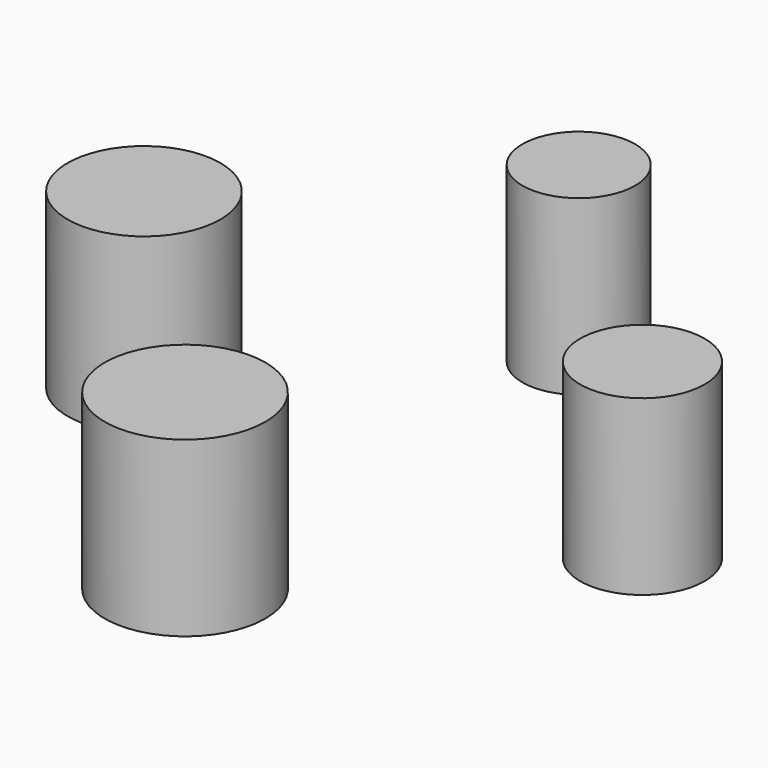
from build123d import *

# Parameters (mm, degrees)
F2_R     = 9.1214460024
F3_DEPTH = 25.4
F4_R     = 11.2110594619
F5_DEPTH = 25.4
F6_R     = 11.7851409997
F7_DEPTH = 25.4
F6_R_2   = 8.2576202632


# Not quite as in the source:
# - the program builds the solid bodies; features that only make, move or delete a surface that nothing else refers to are left out


with BuildPart() as f3:
    # F2 (on Top) → F3 (new body)
    with BuildSketch(Plane.XY):
        with Locations((36.1533612013, 0)):
            Circle(F2_R)
    extrude(amount=F3_DEPTH)


with BuildPart() as f5:
    # F4 (on Top) → F5 (new body)
    with BuildSketch(Plane.XY):
        with Locations((-34.8000079393, -2.6808977127)):
            Circle(F4_R)
    extrude(amount=F5_DEPTH)


with BuildPart() as f7:
    # F6 (on Top) → F7 (new body)
    with BuildSketch(Plane.XY):
        with Locations((0, -38.6552363634)):
            Circle(F6_R)
    extrude(amount=F7_DEPTH)


with BuildPart() as f7b:
    # F6 (on Top) → F7, piece 2 (new body)
    with BuildSketch(Plane.XY):
        with Locations((0, 33.5225760937)):
            Circle(F6_R_2)
    extrude(amount=F7_DEPTH)


solid = Compound([f3.part, f5.part, f7.part, f7b.part])
